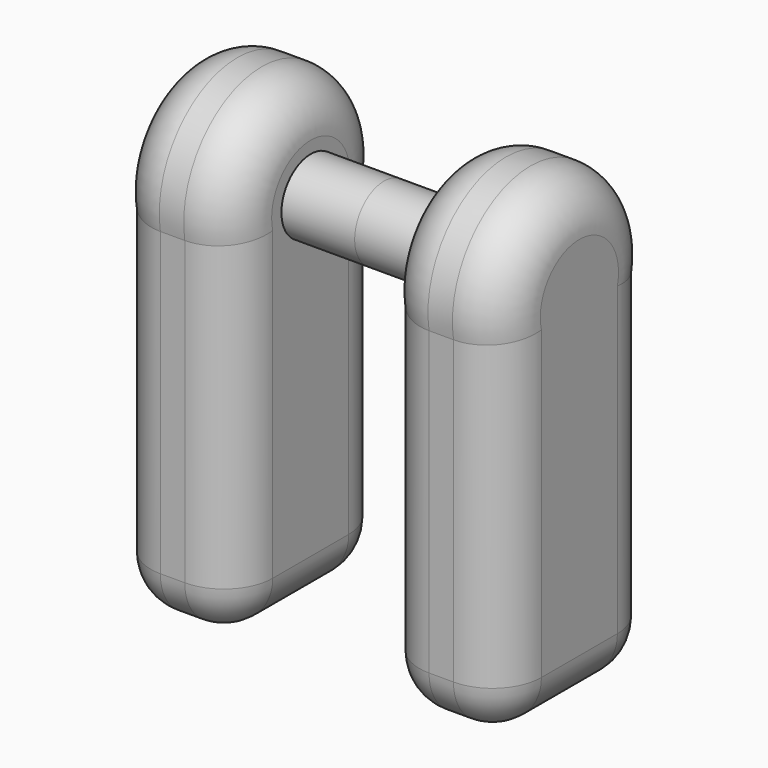
from build123d import *

# Parameters (mm, degrees)
F0_R     = 1.5
F1_DEPTH = 3
F2_R     = 4
F3_W     = 7.888094809
F3_H     = 15
F4_DEPTH = 5
F5_R     = 2
F6_R     = 1.99999


# Not quite as in the source:
# - a fillet or chamfer is up to 0.001 mm smaller than in the source, because OpenCascade refuses the exact size


with BuildPart() as f1:
    # F0 (on Right) → F1 (new body)
    with BuildSketch(Plane.YZ):
        Circle(F0_R)
    extrude(amount=F1_DEPTH)

    # F2 (on Right) + F3 (on Right) → F4 (join)
    with BuildSketch(Plane.YZ):
        Circle(F2_R)
    with BuildSketch(Plane.YZ):
        with Locations((0, -7.5)):
            Rectangle(F3_W, F3_H)
    extrude(amount=-F4_DEPTH)

    # F5
    f5_edges = [f1.edges().sort_by_distance(p)[0] for p in [
        (-5, -3.944047, -7.83335),
        (0, -3.944047, -7.83335),
        (0, 3.944047, -7.83335),
        (-5, 3.944047, -7.83335),
        (-2.5, 3.944047, -15),
        (-5, 0, -15),
        (-2.5, -3.944047, -15),
        (0, 0, -15),
    ]]
    fillet(f5_edges, radius=F5_R)

    # F6 (radius 2 in the source; OpenCascade refuses exactly that, so slightly less here)
    f6_edges = [f1.edges().sort_by_distance(p)[0] for p in [
        (-5, 0, 4),
        (0, 0, 4),
    ]]
    fillet(f6_edges, radius=F6_R)


with BuildPart() as f7_1:
    # F7: instance of F1
    add(f1.part.mirror(Plane.YZ.offset(3)))


solid = Compound([f1.part, f7_1.part])
